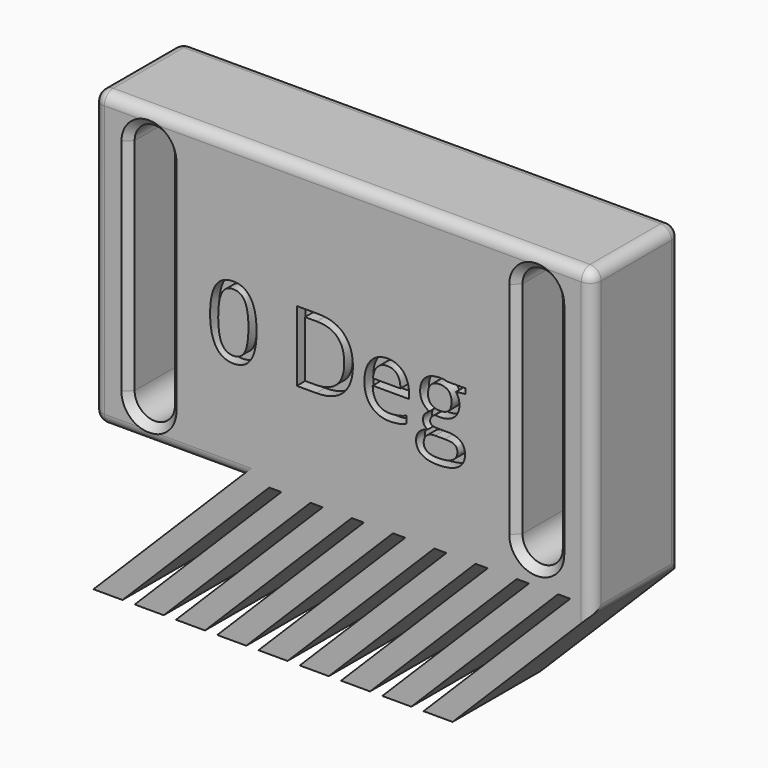
from build123d import *

# Parameters (mm, degrees)
F1_DEPTH     = 15
F2_SIZE      = 1
F3_T1_DEPTH  = 70.25
F3_T3_DEPTH  = 47.5
F3_T5_DEPTH  = 43.2097979746
F3_T7_DEPTH  = 12
F3_T9_DEPTH  = 18.1066017178
F3_S13_W     = 1.5
F3_S13_H     = 1.5
F3_T14_DEPTH = 1.5
F3_S19_W     = 1.5
F3_S19_H     = 1.5
F3_T20_DEPTH = 1.5
F3_T26_DEPTH = 27.5
F3_T31_DEPTH = 27.5
F4_T1_DEPTH  = 12
F4_S5_W      = 1.5
F4_S5_H      = 1.5
F4_T6_DEPTH  = 1.5
F4_S11_W     = 1.5
F4_S11_H     = 1.5
F4_T12_DEPTH = 1.5
F4_S17_W     = 1.5
F4_S17_H     = 1.5
F4_T18_DEPTH = 1.5
F4_S23_W     = 1.5
F4_S23_H     = 1.5
F4_T24_DEPTH = 1.5
F5_TEXT_SIZE = 13.4239125247
F6_DEPTH     = 1.5


# Not quite as in the source:
# - a fillet or chamfer that OpenCascade refuses, or shapes differently, is made with other operations: its cross-section is extruded or revolved along the edge and cut away or added
# - Text() gives the source's letters only with a copy of the font that has no kerning and outlines rounded to 1/6400 em; it was checked with that copy


with BuildPart() as f1:
    # F0 (on Front) → F1 (new body)
    with BuildSketch(Plane.XZ):
        Polygon((34, -10.9597979746), (34, 30), (-34, 30), (-34, -10), (-14, -10), (-34, -30), (-30.0402020254, -30), (-10.0402020254, -10), (-8.375, -10), (-28.375, -30), (-24.4152020254, -30), (-4.4152020254, -10), (-2.75, -10), (-22.75, -30), (-18.7902020254, -30), (1.2097979746, -10), (2.875, -10), (-17.125, -30), (-13.1652020254, -30), (6.8347979746, -10), (8.5, -10), (-11.5, -30), (-7.5402020254, -30), (12.4597979746, -10), (14.125, -10), (-5.875, -30), (-1.9152020254, -30), (18.0847979746, -10), (19.75, -10), (-0.25, -30), (3.7097979746, -30), (23.7097979746, -10), (25.375, -10), (5.375, -30), (9.3347979746, -30), (29.3347979746, -10), (31, -10), (11, -30), (14.9597979746, -30), align=None)
        with BuildLine():
            Line((-29.1851401776, -5), (-29.1851401776, 25))
            ThreePointArc((-29.1851401776, 25), (-26.4351401776, 27.75), (-23.6851401776, 25))
            Line((-23.6851401776, 25), (-23.6851401776, -5))
            ThreePointArc((-23.6851401776, -5), (-26.4351401776, -7.75), (-29.1851401776, -5))
        make_face(mode=Mode.SUBTRACT)
        with BuildLine():
            Line((23.6851401776, -5), (23.6851401776, 25))
            ThreePointArc((23.6851401776, 25), (26.4351401776, 27.75), (29.1851401776, 25))
            Line((29.1851401776, 25), (29.1851401776, -5))
            ThreePointArc((29.1851401776, -5), (26.4351401776, -7.75), (23.6851401776, -5))
        make_face(mode=Mode.SUBTRACT)
    extrude(amount=F1_DEPTH)

    # F2
    f2_edges = [f1.edges().sort_by_distance(p)[0] for p in [
        (-29.18514, -15, 10),
        (-23.68514, 0, 10),
        (29.18514, 0, 10),
        (29.18514, -15, 10),
        (-29.18514, 0, 10),
        (-26.43514, 0, 27.75),
        (-26.43514, -15, 27.75),
        (-23.68514, -15, 10),
        (-26.43514, 0, -7.75),
        (-26.43514, -15, -7.75),
        (26.43514, 0, -7.75),
        (26.43514, -15, -7.75),
        (23.68514, 0, 10),
        (23.68514, -15, 10),
        (26.43514, 0, 27.75),
        (26.43514, -15, 27.75),
    ]]
    chamfer(f2_edges, length=F2_SIZE)

    # F3: fillet of radius 1.5 on 10 edges, made by hand

    # F3_s2 → F3_t1 (cut)
    with BuildSketch(Plane.YZ.offset(-37.75)):
        with BuildLine():
            ThreePointArc((-15, 28.5), (-14.5606601718, 29.5606601718), (-13.5, 30))
            Line((-13.5, 30), (-15, 30))
            Line((-15, 30), (-15, 28.5))
        make_face()
        with BuildLine():
            ThreePointArc((0, 28.5), (-0.4393398282, 29.5606601718), (-1.5, 30))
            Line((-1.5, 30), (0, 30))
            Line((0, 30), (0, 28.5))
        make_face()
    extrude(amount=F3_T1_DEPTH, mode=Mode.SUBTRACT)

    # F3_s4 → F3_t3 (cut)
    with BuildSketch(Plane.XY.offset(-13.75)):
        with BuildLine():
            ThreePointArc((-32.5, -15), (-33.5606601718, -14.5606601718), (-34, -13.5))
            Line((-34, -13.5), (-34, -15))
            Line((-34, -15), (-32.5, -15))
        make_face()
        with BuildLine():
            ThreePointArc((-32.5, 0), (-33.5606601718, -0.4393398282), (-34, -1.5))
            Line((-34, -1.5), (-34, 0))
            Line((-34, 0), (-32.5, 0))
        make_face()
    extrude(amount=F3_T3_DEPTH, mode=Mode.SUBTRACT)

    # F3_s6 → F3_t5 (cut)
    with BuildSketch(Plane.XY.offset(-14.7097979746)):
        with BuildLine():
            ThreePointArc((32.5, -15), (33.5606601718, -14.5606601718), (34, -13.5))
            Line((34, -13.5), (34, -15))
            Line((34, -15), (32.5, -15))
        make_face()
        with BuildLine():
            ThreePointArc((32.5, 0), (33.5606601718, -0.4393398282), (34, -1.5))
            Line((34, -1.5), (34, 0))
            Line((34, 0), (32.5, 0))
        make_face()
    extrude(amount=F3_T5_DEPTH, mode=Mode.SUBTRACT)

    # F3_s8 → F3_t7 (cut)
    with BuildSketch(Plane.XZ.offset(1.5)):
        with BuildLine():
            ThreePointArc((34, 28.5), (33.5606601718, 29.5606601718), (32.5, 30))
            Line((32.5, 30), (34, 30))
            Line((34, 30), (34, 28.5))
        make_face()
    extrude(amount=F3_T7_DEPTH, mode=Mode.SUBTRACT)

    # F3_s10 → F3_t9 (cut)
    with BuildSketch(Plane.XZ.offset(-1.5533008589)):
        with BuildLine():
            ThreePointArc((33.5606601718, -11.3991378029), (33.8858192988, -10.9125027796), (34, -10.3384776311))
            Line((34, -10.3384776311), (34, -10.9597979746))
            Line((34, -10.9597979746), (33.5606601718, -11.3991378029))
        make_face()
    extrude(amount=F3_T9_DEPTH, mode=Mode.SUBTRACT)


with BuildPart() as f3_tool12:
    # F3_s13 → F3_t14 (new body)
    with BuildSketch(Plane.XZ.offset(13.5)):
        with Locations((33.25, 29.25)):
            Rectangle(F3_S13_W, F3_S13_H)
    extrude(amount=F3_T14_DEPTH)

    # F3_s15 → F3_t16 (revolve, cut)
    with BuildSketch(Plane(origin=(32.5, -13.5, 28.5), x_dir=(-0.7071067812, 0, -0.7071067812), z_dir=(-0.7071067812, 0, 0.7071067812))):
        with BuildLine():
            ThreePointArc((0, -1.5), (1.5, 0), (0, 1.5))
            Line((0, 1.5), (0, -1.5))
        make_face()
    revolve(axis=Axis((32.5, -13.5, 28.5), (0, -1, 0)), mode=Mode.SUBTRACT)


with BuildPart() as f1_1:
    add(f1.part)

    # F3_t11: cut F3_tool12
    add(f3_tool12.part, mode=Mode.SUBTRACT)


with BuildPart() as f3_tool18:
    # F3_s19 → F3_t20 (new body)
    with BuildSketch(Plane.XZ.offset(1.5)):
        with Locations((33.25, 29.25)):
            Rectangle(F3_S19_W, F3_S19_H)
    extrude(amount=-F3_T20_DEPTH)

    # F3_s21 → F3_t22 (revolve, cut)
    with BuildSketch(Plane(origin=(32.5, -1.5, 28.5), x_dir=(-0.7071067812, 0, -0.7071067812), z_dir=(0.7071067812, 0, -0.7071067812))):
        with BuildLine():
            ThreePointArc((0, -1.5), (1.5, 0), (0, 1.5))
            Line((0, 1.5), (0, -1.5))
        make_face()
    revolve(axis=Axis((32.5, -1.5, 28.5), (0, 1, 0)), mode=Mode.SUBTRACT)


with BuildPart() as f1_2:
    add(f1_1.part)

    # F3_t17: cut F3_tool18
    add(f3_tool18.part, mode=Mode.SUBTRACT)


with BuildPart() as f3_tool24:
    # F3_s25 → F3_t26 (new body)
    with BuildSketch(Plane.YZ.offset(-37.75)):
        with BuildLine():
            ThreePointArc((-15, -8.5), (-14.5606601718, -9.5606601718), (-13.5, -10))
            Line((-13.5, -10), (-15, -10))
            Line((-15, -10), (-15, -8.5))
        make_face()
    extrude(amount=F3_T26_DEPTH)

    split(bisect_by=Plane(origin=(-2, 0, 2), x_dir=(0, 1, 0), z_dir=(-0.7071067812, 0, 0.7071067812)), keep=Keep.TOP)


with BuildPart() as f1_3:
    add(f1_2.part)

    # F3_t23: cut F3_tool24
    add(f3_tool24.part, mode=Mode.SUBTRACT)


with BuildPart() as f3_tool29:
    # F3_s30 → F3_t31 (new body)
    with BuildSketch(Plane.YZ.offset(-37.75)):
        with BuildLine():
            ThreePointArc((0, -8.5), (-0.4393398282, -9.5606601718), (-1.5, -10))
            Line((-1.5, -10), (0, -10))
            Line((0, -10), (0, -8.5))
        make_face()
    extrude(amount=F3_T31_DEPTH)

    split(bisect_by=Plane(origin=(-2, 0, 2), x_dir=(0, 1, 0), z_dir=(-0.7071067812, 0, 0.7071067812)), keep=Keep.TOP)


with BuildPart() as f1_4:
    add(f1_3.part)

    # F3_t28: cut F3_tool29
    add(f3_tool29.part, mode=Mode.SUBTRACT)

    # F4: fillet of radius 1.5 on 2 edges, made by hand

    # F4_s2 → F4_t1 (cut)
    with BuildSketch(Plane.XZ.offset(1.5)):
        with BuildLine():
            ThreePointArc((-32.5, -10), (-33.5606601718, -9.5606601718), (-34, -8.5))
            Line((-34, -8.5), (-34, -10))
            Line((-34, -10), (-32.5, -10))
        make_face()
        with BuildLine():
            ThreePointArc((-34, 28.5), (-33.5606601718, 29.5606601718), (-32.5, 30))
            Line((-32.5, 30), (-34, 30))
            Line((-34, 30), (-34, 28.5))
        make_face()
    extrude(amount=F4_T1_DEPTH, mode=Mode.SUBTRACT)


with BuildPart() as f4_tool4:
    # F4_s5 → F4_t6 (new body)
    with BuildSketch(Plane.YZ.offset(-32.5)):
        with Locations((-0.75, 29.25)):
            Rectangle(F4_S5_W, F4_S5_H)
    extrude(amount=-F4_T6_DEPTH)

    # F4_s7 → F4_t8 (revolve, cut)
    with BuildSketch(Plane(origin=(-32.5, -1.5, 28.5), x_dir=(0, -0.7071067812, -0.7071067812), z_dir=(0, 0.7071067812, -0.7071067812))):
        with BuildLine():
            ThreePointArc((0, -1.5), (1.5, 0), (0, 1.5))
            Line((0, 1.5), (0, -1.5))
        make_face()
    revolve(axis=Axis((-32.5, -1.5, 28.5), (-1, 0, 0)), mode=Mode.SUBTRACT)


with BuildPart() as f1_5:
    add(f1_4.part)

    # F4_t3: cut F4_tool4
    add(f4_tool4.part, mode=Mode.SUBTRACT)


with BuildPart() as f4_tool10:
    # F4_s11 → F4_t12 (new body)
    with BuildSketch(Plane.YZ.offset(-32.5)):
        with Locations((-14.25, 29.25)):
            Rectangle(F4_S11_W, F4_S11_H)
    extrude(amount=-F4_T12_DEPTH)

    # F4_s13 → F4_t14 (revolve, cut)
    with BuildSketch(Plane(origin=(-32.5, -13.5, 28.5), x_dir=(0, 0.7071067812, -0.7071067812), z_dir=(0, 0.7071067812, 0.7071067812))):
        with BuildLine():
            ThreePointArc((0, -1.5), (1.5, 0), (0, 1.5))
            Line((0, 1.5), (0, -1.5))
        make_face()
    revolve(axis=Axis((-32.5, -13.5, 28.5), (-1, 0, 0)), mode=Mode.SUBTRACT)


with BuildPart() as f1_6:
    add(f1_5.part)

    # F4_t9: cut F4_tool10
    add(f4_tool10.part, mode=Mode.SUBTRACT)


with BuildPart() as f4_tool16:
    # F4_s17 → F4_t18 (new body)
    with BuildSketch(Plane.XY.offset(-8.5)):
        with Locations((-33.25, -0.75)):
            Rectangle(F4_S17_W, F4_S17_H)
    extrude(amount=-F4_T18_DEPTH)

    # F4_s19 → F4_t20 (revolve, cut)
    with BuildSketch(Plane(origin=(-32.5, -1.5, -8.5), x_dir=(0.7071067812, -0.7071067812, 0), z_dir=(0.7071067812, 0.7071067812, 0))):
        with BuildLine():
            ThreePointArc((0, -1.5), (1.5, 0), (0, 1.5))
            Line((0, 1.5), (0, -1.5))
        make_face()
    revolve(axis=Axis((-32.5, -1.5, -8.5), (0, 0, -1)), mode=Mode.SUBTRACT)


with BuildPart() as f1_7:
    add(f1_6.part)

    # F4_t15: cut F4_tool16
    add(f4_tool16.part, mode=Mode.SUBTRACT)


with BuildPart() as f4_tool22:
    # F4_s23 → F4_t24 (new body)
    with BuildSketch(Plane.XY.offset(-8.5)):
        with Locations((-33.25, -14.25)):
            Rectangle(F4_S23_W, F4_S23_H)
    extrude(amount=-F4_T24_DEPTH)

    # F4_s25 → F4_t26 (revolve, cut)
    with BuildSketch(Plane(origin=(-32.5, -13.5, -8.5), x_dir=(0.7071067812, 0.7071067812, 0), z_dir=(-0.7071067812, 0.7071067812, 0))):
        with BuildLine():
            ThreePointArc((0, -1.5), (1.5, 0), (0, 1.5))
            Line((0, 1.5), (0, -1.5))
        make_face()
    revolve(axis=Axis((-32.5, -13.5, -8.5), (0, 0, -1)), mode=Mode.SUBTRACT)


with BuildPart() as f1_8:
    add(f1_7.part)

    # F4_t21: cut F4_tool22
    add(f4_tool22.part, mode=Mode.SUBTRACT)

    # F5 (on face) → F6 (cut)
    with BuildSketch(Plane.XZ.offset(15)):
        with Locations((-18.7624534592, 3.4236155916)):
            Text('0 Deg', F5_TEXT_SIZE, font='Open Sans', text_align=(TextAlign.LEFT, TextAlign.BOTTOM))
    extrude(amount=-F6_DEPTH, mode=Mode.SUBTRACT)


solid = f1_8.part
